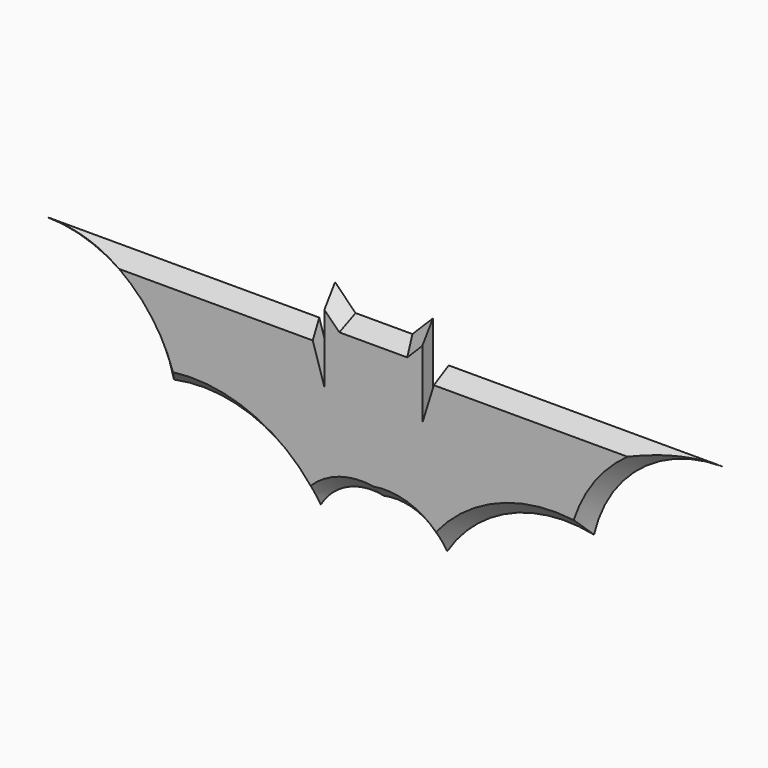
from build123d import *

# Parameters (mm, degrees)
F1_DEPTH = 2.54
F2_SIZE  = 2.53999


# Not quite as in the source:
# - a fillet or chamfer is up to 0.001 mm smaller than in the source, because OpenCascade refuses the exact size


with BuildPart() as f1:
    # F0 (on Front) → F1 (new body)
    with BuildSketch(Plane.XZ):
        with BuildLine():
            Line((-12.3092299327, 19.36452277), (-64.2481818795, 19.36452277))
            ThreePointArc((-64.2481818795, 19.36452277), (-48.7050050326, 13.9320089842), (-39.9299450219, 0))
            ThreePointArc((-39.9299450219, 0), (-24.1018123493, -1.5321631259), (-12.0090059936, -11.8588926271))
            ThreePointArc((-12.0090059936, -11.8588926271), (-6.881876251, -7.2071480524), (0, -6.4548407681))
            ThreePointArc((0, -6.4548407681), (6.881876251, -7.2071480524), (12.0090059936, -11.8588926271))
            ThreePointArc((12.0090059936, -11.8588926271), (24.1018123493, -1.5321631259), (39.9299450219, 0))
            ThreePointArc((39.9299450219, 0), (48.7050050326, 13.9320089842), (64.2481818795, 19.36452277))
            Line((64.2481818795, 19.36452277), (12.3092299327, 19.36452277))
            Line((12.3092299327, 19.36452277), (9.3069793656, 9.7573176026))
            Line((9.3069793656, 9.7573176026), (9.3069793656, 26.2697003782))
            Line((9.3069793656, 26.2697003782), (5.4040518589, 22.3667733371))
            Line((5.4040518589, 22.3667733371), (0, 22.3667733371))
            Line((0, 22.3667733371), (-5.4040518589, 22.3667733371))
            Line((-5.4040518589, 22.3667733371), (-9.3069793656, 26.2697003782))
            Line((-9.3069793656, 26.2697003782), (-9.3069793656, 9.7573176026))
            Line((-9.3069793656, 9.7573176026), (-12.3092299327, 19.36452277))
        make_face()
    extrude(amount=F1_DEPTH)

    # F2 (size 2.54 in the source; OpenCascade refuses exactly that, so slightly less here)
    f2_edges = [f1.edges().sort_by_distance(p)[0] for p in [
        (-38.278706, -2.54, 19.364523),
        (38.278706, -2.54, 19.364523),
        (48.705005, -2.54, 13.932009),
        (24.101812, -2.54, -1.532163),
        (6.881876, -2.54, -7.207148),
        (-6.881876, -2.54, -7.207148),
        (-24.101812, -2.54, -1.532163),
        (-48.705005, -2.54, 13.932009),
        (-7.355516, -2.54, 24.318237),
        (0, -2.54, 22.366773),
        (7.355516, -2.54, 24.318237),
    ]]
    chamfer(f2_edges, length=F2_SIZE)


solid = f1.part
